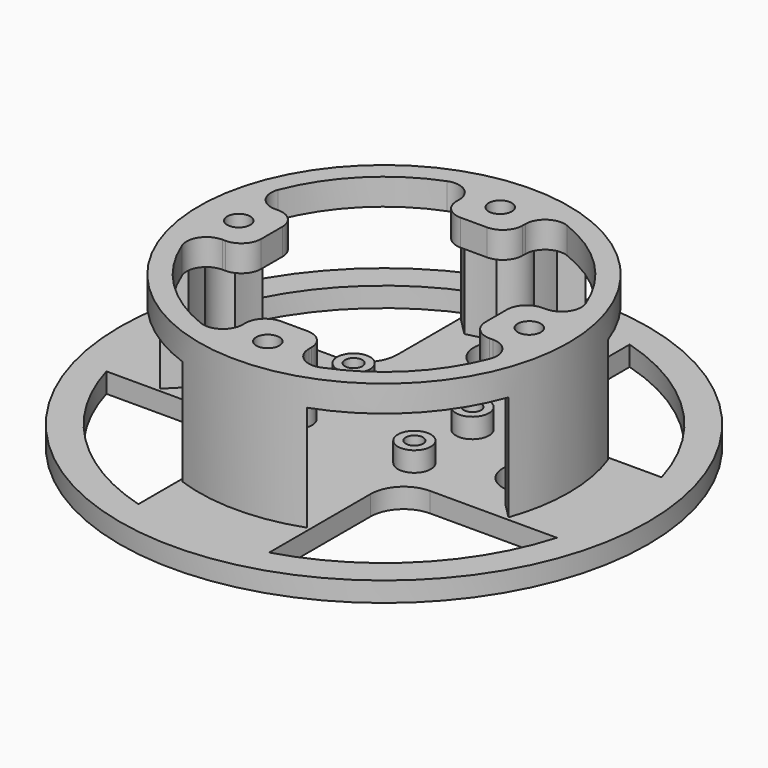
from build123d import *

# Parameters (mm, degrees)
F0_R        = 40
F1_DEPTH    = 3
F2_R        = 28
F3_DEPTH    = 16
F4_R        = 25
F5_DEPTH    = 16
F6_R        = 28
F6_R_2      = 1.75
F7_DEPTH    = 4
F8_T1_DEPTH = 4
F8_T3_DEPTH = 19
F9_R        = 4
F10_DEPTH   = 19
F13_W       = 24
F13_H       = 16
F14_DEPTH   = 84.5695424949
F16_W       = 24
F16_H       = 16
F17_DEPTH   = 84.5695424949
F18_R       = 1.3
F19_DEPTH   = 3.001
F20_R       = 2.5
F20_R_2     = 1.3088878735
F21_DEPTH   = 3
F23_DEPTH   = 3
F24_R       = 5


# Not quite as in the source:
# - a fillet or chamfer that OpenCascade refuses, or shapes differently, is made with other operations: its cross-section is extruded or revolved along the edge and cut away or added
# - an extrude ends at something that could not be found from the text; its depth is read off the source's solid


with BuildPart() as f1:
    # F0 (on Top) → F1 (new body)
    with BuildSketch(Plane.XY):
        Circle(F0_R)
    extrude(amount=F1_DEPTH)

    # F2 (on face) → F3 (join)
    with BuildSketch(Plane.XY.offset(3)):
        Circle(F2_R)
    extrude(amount=F3_DEPTH)

    # F4 (on face) → F5 (cut)
    with BuildSketch(Plane.XY.offset(19)):
        Circle(F4_R)
    extrude(amount=-F5_DEPTH, mode=Mode.SUBTRACT)

    # F6 (on face) → F7 (join)
    with BuildSketch(Plane.XY.offset(19)):
        Circle(F6_R)
        with BuildLine():
            ThreePointArc((-5, 24.4948974278), (0, 25), (5, 24.4948974278))
            ThreePointArc((5, 24.4948974278), (17.6776695297, 17.6776695297), (24.4948974278, 5))
            ThreePointArc((24.4948974278, 5), (24.8734038251, 2.5127240501), (25, 0))
            ThreePointArc((25, 0), (24.8734038251, -2.5127240501), (24.4948974278, -5))
            ThreePointArc((24.4948974278, -5), (17.6776695297, -17.6776695297), (5, -24.4948974278))
            ThreePointArc((5, -24.4948974278), (0, -25), (-5, -24.4948974278))
            ThreePointArc((-5, -24.4948974278), (-17.6776695297, -17.6776695297), (-24.4948974278, -5))
            ThreePointArc((-24.4948974278, -5), (-25, 0), (-24.4948974278, 5))
            ThreePointArc((-24.4948974278, 5), (-17.6776695297, 17.6776695297), (-5, 24.4948974278))
        make_face(mode=Mode.SUBTRACT)
        with BuildLine():
            Line((-17, 5), (-24.4948974278, 5))
            ThreePointArc((-24.4948974278, 5), (-25, 0), (-24.4948974278, -5))
            Line((-24.4948974278, -5), (-17, -5))
            Line((-17, -5), (-17, 5))
        make_face()
        with Locations((-22, 0)):
            Circle(F6_R_2, mode=Mode.SUBTRACT)
        with BuildLine():
            Line((-5, 17), (5, 17))
            Line((5, 17), (5, 24.4948974278))
            ThreePointArc((5, 24.4948974278), (0, 25), (-5, 24.4948974278))
            Line((-5, 24.4948974278), (-5, 17))
        make_face()
        with Locations((0, 22)):
            Circle(F6_R_2, mode=Mode.SUBTRACT)
        with BuildLine():
            ThreePointArc((25, 0), (24.8734038251, 2.5127240501), (24.4948974278, 5))
            Line((24.4948974278, 5), (17, 5))
            Line((17, 5), (17, -5))
            Line((17, -5), (24.4948974278, -5))
            ThreePointArc((24.4948974278, -5), (24.8734038251, -2.5127240501), (25, 0))
        make_face()
        with Locations((22, 0)):
            Circle(F6_R_2, mode=Mode.SUBTRACT)
        with BuildLine():
            Line((-5, -17), (-5, -24.4948974278))
            ThreePointArc((-5, -24.4948974278), (0, -25), (5, -24.4948974278))
            Line((5, -24.4948974278), (5, -17))
            Line((5, -17), (-5, -17))
        make_face()
        with Locations((0, -22)):
            Circle(F6_R_2, mode=Mode.SUBTRACT)
    extrude(amount=F7_DEPTH)

    # F8: fillet of radius 3 on 16 edges, made by hand

    # F8_s2 → F8_t1 (join)
    with BuildSketch(Plane.XY.offset(19)):
        with BuildLine():
            ThreePointArc((9.0909090909, 23.2885244681), (6.3077717755, 22.9710700035), (5, 20.4939015319))
            Line((5, 20.4939015319), (5, 24.4948974278))
            ThreePointArc((5, 24.4948974278), (7.0712278765, 23.9791104155), (9.0909090909, 23.2885244681))
        make_face()
        with BuildLine():
            ThreePointArc((-5, 20.4939015319), (-6.3077717755, 22.9710700035), (-9.0909090909, 23.2885244681))
            ThreePointArc((-9.0909090909, 23.2885244681), (-7.0712278765, 23.9791104155), (-5, 24.4948974278))
            Line((-5, 24.4948974278), (-5, 20.4939015319))
        make_face()
        with BuildLine():
            ThreePointArc((-23.2885244681, 9.0909090909), (-22.9710700035, 6.3077717755), (-20.4939015319, 5))
            Line((-20.4939015319, 5), (-24.4948974278, 5))
            ThreePointArc((-24.4948974278, 5), (-23.9791104155, 7.0712278765), (-23.2885244681, 9.0909090909))
        make_face()
        with BuildLine():
            ThreePointArc((-23.2885244681, -9.0909090909), (-22.9710700035, -6.3077717755), (-20.4939015319, -5))
            Line((-20.4939015319, -5), (-24.4948974278, -5))
            ThreePointArc((-24.4948974278, -5), (-23.9791104155, -7.0712278765), (-23.2885244681, -9.0909090909))
        make_face()
        with BuildLine():
            ThreePointArc((20.4939015319, 5), (22.9710700035, 6.3077717755), (23.2885244681, 9.0909090909))
            ThreePointArc((23.2885244681, 9.0909090909), (23.9791104155, 7.0712278765), (24.4948974278, 5))
            Line((24.4948974278, 5), (20.4939015319, 5))
        make_face()
        with BuildLine():
            ThreePointArc((23.2885244681, -9.0909090909), (22.9710700035, -6.3077717755), (20.4939015319, -5))
            Line((20.4939015319, -5), (24.4948974278, -5))
            ThreePointArc((24.4948974278, -5), (23.9791104155, -7.0712278765), (23.2885244681, -9.0909090909))
        make_face()
        with BuildLine():
            ThreePointArc((-9.0909090909, -23.2885244681), (-6.3077717755, -22.9710700035), (-5, -20.4939015319))
            Line((-5, -20.4939015319), (-5, -24.4948974278))
            ThreePointArc((-5, -24.4948974278), (-7.0712278765, -23.9791104155), (-9.0909090909, -23.2885244681))
        make_face()
        with BuildLine():
            ThreePointArc((5, -20.4939015319), (6.3077717755, -22.9710700035), (9.0909090909, -23.2885244681))
            ThreePointArc((9.0909090909, -23.2885244681), (7.0712278765, -23.9791104155), (5, -24.4948974278))
            Line((5, -24.4948974278), (5, -20.4939015319))
        make_face()
    extrude(amount=F8_T1_DEPTH)

    # F8_s4 → F8_t3 (cut)
    with BuildSketch(Plane.XY.offset(11.5)):
        with BuildLine():
            ThreePointArc((-17, -2), (-17.8786796564, -4.1213203436), (-20, -5))
            Line((-20, -5), (-17, -5))
            Line((-17, -5), (-17, -2))
        make_face()
        with BuildLine():
            ThreePointArc((-20, 5), (-17.8786796564, 4.1213203436), (-17, 2))
            Line((-17, 2), (-17, 5))
            Line((-17, 5), (-20, 5))
        make_face()
        with BuildLine():
            ThreePointArc((-2, 17), (-4.1213203436, 17.8786796564), (-5, 20))
            Line((-5, 20), (-5, 17))
            Line((-5, 17), (-2, 17))
        make_face()
        with BuildLine():
            ThreePointArc((5, 20), (4.1213203436, 17.8786796564), (2, 17))
            Line((2, 17), (5, 17))
            Line((5, 17), (5, 20))
        make_face()
        with BuildLine():
            ThreePointArc((20, -5), (17.8786796564, -4.1213203436), (17, -2))
            Line((17, -2), (17, -5))
            Line((17, -5), (20, -5))
        make_face()
        with BuildLine():
            ThreePointArc((17, 2), (17.8786796564, 4.1213203436), (20, 5))
            Line((20, 5), (17, 5))
            Line((17, 5), (17, 2))
        make_face()
        with BuildLine():
            ThreePointArc((2, -17), (4.1213203436, -17.8786796564), (5, -20))
            Line((5, -20), (5, -17))
            Line((5, -17), (2, -17))
        make_face()
        with BuildLine():
            ThreePointArc((-5, -20), (-4.1213203436, -17.8786796564), (-2, -17))
            Line((-2, -17), (-5, -17))
            Line((-5, -17), (-5, -20))
        make_face()
    extrude(amount=F8_T3_DEPTH, mode=Mode.SUBTRACT)

    # F9 (on face) → F10 (cut, through all)
    with BuildSketch(Plane(origin=(0, 0, 0), x_dir=(1, 0, 0), z_dir=(0, 0, -1))):
        with Locations((0, 22)):
            Circle(F9_R)
        with Locations((-22, 0)):
            Circle(F9_R)
        with Locations((0, -22)):
            Circle(F9_R)
        with Locations((22, 0)):
            Circle(F9_R)
    extrude(amount=-F10_DEPTH, mode=Mode.SUBTRACT)

    # F13 (on line) → F14 (cut, through all)
    with BuildSketch(Plane(origin=(-19.7989898732, -19.7989898732, 0), x_dir=(0.7071067812, -0.7071067812, 0), z_dir=(-0.7071067812, -0.7071067812, 0))):
        with Locations((0, 11)):
            Rectangle(F13_W, F13_H)
    extrude(amount=-F14_DEPTH, mode=Mode.SUBTRACT)

    # F16 (on line) → F17 (cut, through all)
    with BuildSketch(Plane(origin=(-19.7989898732, 19.7989898732, 0), x_dir=(-0.7071067812, -0.7071067812, 0), z_dir=(-0.7071067812, 0.7071067812, 0))):
        with Locations((0, 11)):
            Rectangle(F16_W, F16_H)
    extrude(amount=-F17_DEPTH, mode=Mode.SUBTRACT)

    # F18 (on face) → F19 (cut, through all)
    with BuildSketch(Plane.XY.offset(3)):
        with Locations((-9, 5.5)):
            Circle(F18_R)
        with Locations((9, 5.5)):
            Circle(F18_R)
        with Locations((9, -5.5)):
            Circle(F18_R)
        with Locations((-9, -5.5)):
            Circle(F18_R)
    extrude(amount=-F19_DEPTH, mode=Mode.SUBTRACT)

    # F20 (on face) → F21 (join)
    with BuildSketch(Plane.XY.offset(3)):
        with Locations((-9, 5.5)):
            Circle(F20_R)
        with Locations((-9, 5.5)):
            Circle(F20_R_2, mode=Mode.SUBTRACT)
        with Locations((9, 5.5)):
            Circle(F20_R)
        with Locations((9, 5.5)):
            Circle(F20_R_2, mode=Mode.SUBTRACT)
        with Locations((-9, -5.5)):
            Circle(F20_R)
        with Locations((-9, -5.5)):
            Circle(F20_R_2, mode=Mode.SUBTRACT)
        with Locations((9, -5.5)):
            Circle(F20_R)
        with Locations((9, -5.5)):
            Circle(F20_R_2, mode=Mode.SUBTRACT)
    extrude(amount=F21_DEPTH)

    # F22 (on face) → F23 (cut, through all)
    with BuildSketch(Plane(origin=(0, 0, 0), x_dir=(1, 0, 0), z_dir=(0, 0, -1))):
        with BuildLine():
            Line((-9.9123141263, 9.9123141263), (-9.9123141263, 34.1129360408))
            ThreePointArc((-9.9123141263, 34.1129360408), (-18.0837856402, 30.5765117954), (-25.1191796906, 25.1191796906))
            Line((-25.1191796906, 25.1191796906), (-9.9123141263, 9.9123141263))
        make_face()
        with BuildLine():
            Line((-9.9123141263, 9.9123141263), (-25.1191796906, 25.1191796906))
            ThreePointArc((-25.1191796906, 25.1191796906), (-30.5765117954, 18.0837856402), (-34.1129360408, 9.9123141263))
            Line((-34.1129360408, 9.9123141263), (-9.9123141263, 9.9123141263))
        make_face()
        with BuildLine():
            Line((9.9123141263, 9.9123141263), (34.1129360408, 9.9123141263))
            ThreePointArc((34.1129360408, 9.9123141263), (25.1191796906, 25.1191796906), (9.9123141263, 34.1129360408))
            Line((9.9123141263, 34.1129360408), (9.9123141263, 9.9123141263))
        make_face()
        with BuildLine():
            ThreePointArc((9.9123141263, -34.1129360408), (25.1191796906, -25.1191796906), (34.1129360408, -9.9123141263))
            Line((34.1129360408, -9.9123141263), (9.9123141263, -9.9123141263))
            Line((9.9123141263, -9.9123141263), (9.9123141263, -34.1129360408))
        make_face()
        with BuildLine():
            ThreePointArc((-34.1129360408, -9.9123141263), (-25.1191796906, -25.1191796906), (-9.9123141263, -34.1129360408))
            Line((-9.9123141263, -34.1129360408), (-9.9123141263, -9.9123141263))
            Line((-9.9123141263, -9.9123141263), (-34.1129360408, -9.9123141263))
        make_face()
    extrude(amount=-F23_DEPTH, mode=Mode.SUBTRACT)

    # F24
    f24_edges = [f1.edges().sort_by_distance(p)[0] for p in [
        (9.912314, 9.912314, 1.5),
        (9.912314, -9.912314, 1.5),
        (-9.912314, 9.912314, 1.5),
        (-9.912314, -9.912314, 1.5),
    ]]
    fillet(f24_edges, radius=F24_R)


solid = f1.part
